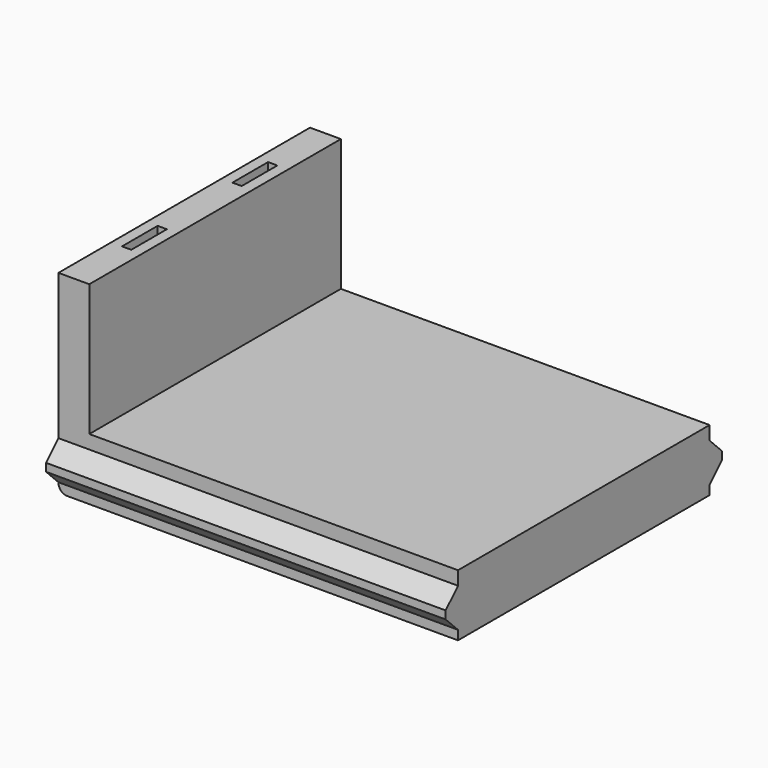
from build123d import *

# Parameters (mm, degrees)
F0_W      = 90.6
F0_H      = 71.3
F1_DEPTH  = 14
F2_W      = 7
F2_H      = 71.3
F3_DEPTH  = 29.9
F5_DEPTH  = 90.6
F7_W      = 2.1
F7_H      = 10.1
F8_DEPTH  = 20.05
F9_R      = 5.04999
F10_R     = 2
F12_DEPTH = 5
F13_R     = 4


# Not quite as in the source:
# - a fillet or chamfer is up to 0.001 mm smaller than in the source, because OpenCascade refuses the exact size


with BuildPart() as f1:
    # F0 (on Top) → F1 (new body)
    with BuildSketch(Plane.XY):
        Rectangle(F0_W, F0_H)
    extrude(amount=F1_DEPTH)

    # F2 (on face) → F3 (join)
    with BuildSketch(Plane.XY.offset(14)):
        with Locations((-41.8, 0)):
            Rectangle(F2_W, F2_H)
    extrude(amount=F3_DEPTH)


with BuildPart() as f5:
    # F4 (on face) → F5 (new body)
    with BuildSketch(Plane.YZ.offset(45.3)):
        Polygon((-39.15, 5.6), (-35.65, 2.1), (-35.65, 10.9), (-39.15, 7.4), align=None)
    extrude(amount=-F5_DEPTH)


with BuildPart() as f5b:
    # F4 (on face) → F5, piece 2 (new body)
    with BuildSketch(Plane.YZ.offset(45.3)):
        Polygon((35.65, 10.9), (35.65, 2.1), (39.15, 5.6), (39.15, 7.4), align=None)
    extrude(amount=-F5_DEPTH)


with BuildPart() as f5_1:
    add(f5.part)

    # F6: union F1, F5b
    add(f1.part)
    add(f5b.part)

    # F7 (on face) → F8 (cut)
    with BuildSketch(Plane.XY.offset(43.9)):
        with Locations((-41.8, -15.65)):
            Rectangle(F7_W, F7_H)
        with Locations((-41.8, 15.65)):
            Rectangle(F7_W, F7_H)
    extrude(amount=-F8_DEPTH, mode=Mode.SUBTRACT)

    # F9 (radius 5.05 in the source; OpenCascade refuses exactly that, so slightly less here)
    f9_edges = [f5_1.edges().sort_by_distance(p)[0] for p in [
        (-41.8, -20.7, 23.85),
        (-41.8, -10.6, 23.85),
        (-41.8, 20.7, 23.85),
        (-41.8, 10.6, 23.85),
    ]]
    fillet(f9_edges, radius=F9_R)

    # F10
    f10_edges = [f5_1.edges().sort_by_distance(p)[0] for p in [
        (-45.3, 0, 0),
    ]]
    fillet(f10_edges, radius=F10_R)

    # F11 (on face) → F12 (cut)
    with BuildSketch(Plane(origin=(0, 0, 0), x_dir=(1, 0, 0), z_dir=(0, 0, -1))):
        with BuildLine():
            Line((-23.3, 28), (-23.3, -28))
            ThreePointArc((-23.3, -28), (-18.3, -33), (-13.3, -28))
            Line((-13.3, -28), (-13.3, 28))
            ThreePointArc((-13.3, 28), (-18.3, 33), (-23.3, 28))
        make_face()
    extrude(amount=-F12_DEPTH, mode=Mode.SUBTRACT)

    # F13
    f13_edges = [f5_1.edges().sort_by_distance(p)[0] for p in [
        (-23.3, 0, 5),
        (-18.3, 33, 5),
        (-13.3, 0, 5),
        (-18.3, -33, 5),
    ]]
    fillet(f13_edges, radius=F13_R)


solid = f5_1.part
